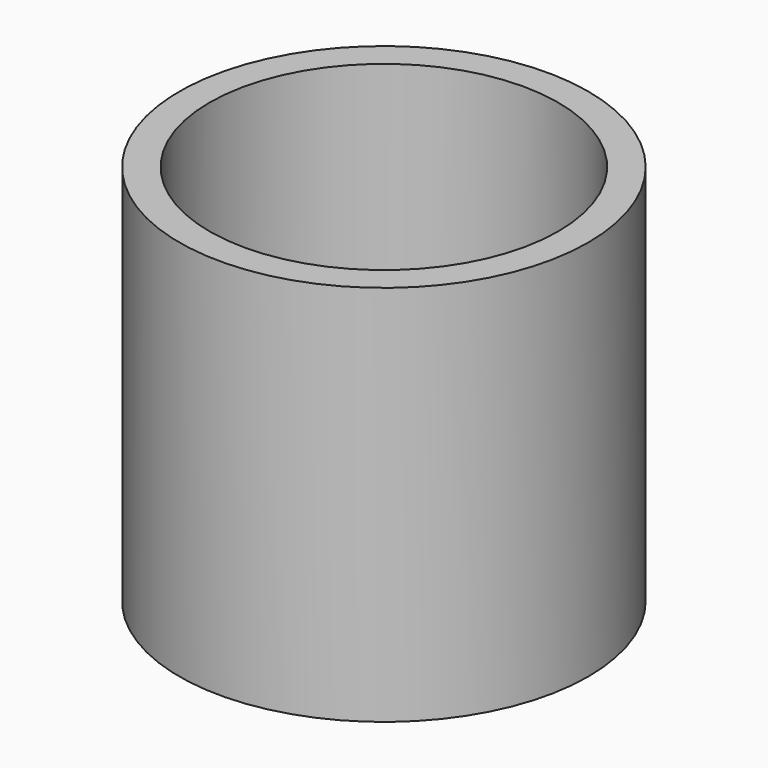
from build123d import *

# Parameters (mm, degrees)
F0_R     = 23.921663712
F0_R_2   = 20.40073985
F1_DEPTH = 44.704
F2_DEPTH = 0.254


# Not quite as in the source:
# - the program builds the solid bodies; features that only make, move or delete a surface that nothing else refers to are left out


with BuildPart() as f1:
    # F0 (on Top) → F1 (new body)
    with BuildSketch(Plane.XY):
        Circle(F0_R)
        Circle(F0_R_2, mode=Mode.SUBTRACT)
    extrude(amount=F1_DEPTH)

    # F0 (on Top) → F2 (join)
    with BuildSketch(Plane.XY):
        Circle(F0_R_2)
    extrude(amount=F2_DEPTH)


solid = f1.part
